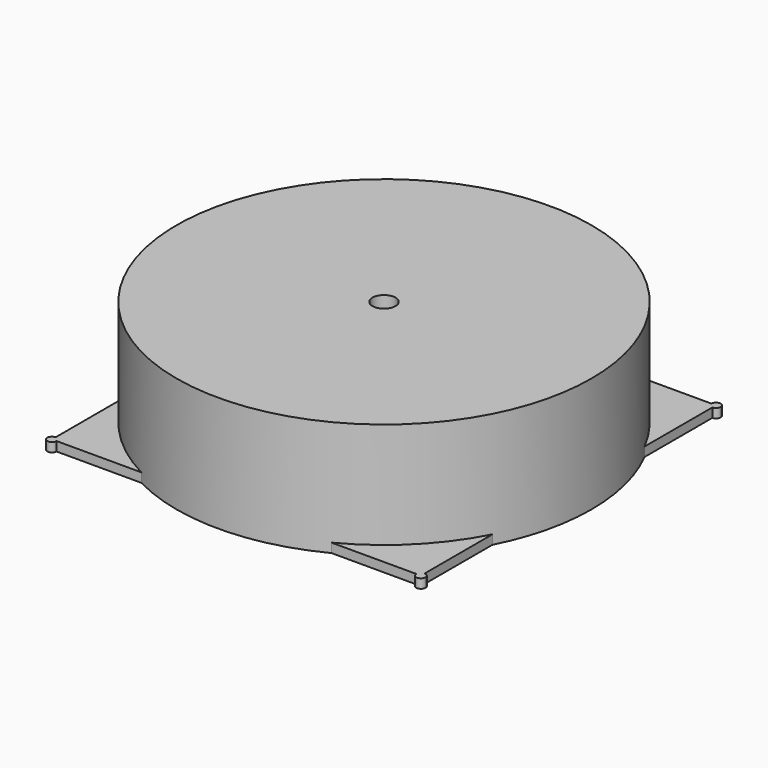
from build123d import *

# Parameters (mm, degrees)
F0_R     = 2.5
F1_DEPTH = 2
F2_DEPTH = 25


# Not quite as in the source:
# - a feature names something its author has since deleted; it is built from what else it names


with BuildPart() as f1:
    # F0 (on Top) → F1 (new body)
    with BuildSketch(Plane.XY):
        with BuildLine():
            ThreePointArc((40, 39), (39.2928932188, 39.2928932188), (39, 40))
            Line((39, 40), (20.6155281281, 40))
            ThreePointArc((20.6155281281, 40), (31.8198051534, 31.8198051534), (40, 20.6155281281))
            Line((40, 20.6155281281), (40, 39))
        make_face()
        with BuildLine():
            ThreePointArc((-40, 20.6155281281), (-31.8198051534, 31.8198051534), (-20.6155281281, 40))
            Line((-20.6155281281, 40), (-39, 40))
            ThreePointArc((-39, 40), (-39.2928932188, 39.2928932188), (-40, 39))
            Line((-40, 39), (-40, 20.6155281281))
        make_face()
        with BuildLine():
            ThreePointArc((-20.6155281281, -40), (-31.8198051534, -31.8198051534), (-40, -20.6155281281))
            Line((-40, -20.6155281281), (-40, -39))
            ThreePointArc((-40, -39), (-39.2928932188, -39.2928932188), (-39, -40))
            Line((-39, -40), (-20.6155281281, -40))
        make_face()
        with BuildLine():
            Line((40, -39), (40, -20.6155281281))
            ThreePointArc((40, -20.6155281281), (31.8198051534, -31.8198051534), (20.6155281281, -40))
            Line((20.6155281281, -40), (39, -40))
            ThreePointArc((39, -40), (39.2928932188, -39.2928932188), (40, -39))
        make_face()
        with BuildLine():
            ThreePointArc((40, 20.6155281281), (31.8198051534, 31.8198051534), (20.6155281281, 40))
            ThreePointArc((20.6155281281, 40), (0, 45), (-20.6155281281, 40))
            ThreePointArc((-20.6155281281, 40), (-31.8198051534, 31.8198051534), (-40, 20.6155281281))
            ThreePointArc((-40, 20.6155281281), (-45, 0), (-40, -20.6155281281))
            ThreePointArc((-40, -20.6155281281), (-31.8198051534, -31.8198051534), (-20.6155281281, -40))
            ThreePointArc((-20.6155281281, -40), (0, -45), (20.6155281281, -40))
            ThreePointArc((20.6155281281, -40), (31.8198051534, -31.8198051534), (40, -20.6155281281))
            ThreePointArc((40, -20.6155281281), (43.7321392113, -10.6066017178), (45, 0))
            ThreePointArc((45, 0), (43.7321392113, 10.6066017178), (40, 20.6155281281))
        make_face()
        Circle(F0_R, mode=Mode.SUBTRACT)
        with BuildLine():
            Line((-40, 40), (-39, 40))
            ThreePointArc((-39, 40), (-40.7071067812, 40.7071067812), (-40, 39))
            Line((-40, 39), (-40, 40))
        make_face()
        with BuildLine():
            ThreePointArc((-40, 39), (-39.2928932188, 39.2928932188), (-39, 40))
            Line((-39, 40), (-40, 40))
            Line((-40, 40), (-40, 39))
        make_face()
        with BuildLine():
            Line((40, 40), (39, 40))
            ThreePointArc((39, 40), (39.2928932188, 39.2928932188), (40, 39))
            Line((40, 39), (40, 40))
        make_face()
        with BuildLine():
            ThreePointArc((40, 39), (40.7071067812, 39.2928932188), (41, 40))
            ThreePointArc((41, 40), (40, 41), (39, 40))
            Line((39, 40), (40, 40))
            Line((40, 40), (40, 39))
        make_face()
        with BuildLine():
            ThreePointArc((41, -40), (40.7071067812, -39.2928932188), (40, -39))
            Line((40, -39), (40, -40))
            Line((40, -40), (39, -40))
            ThreePointArc((39, -40), (40, -41), (41, -40))
        make_face()
        with BuildLine():
            Line((40, -40), (40, -39))
            ThreePointArc((40, -39), (39.2928932188, -39.2928932188), (39, -40))
            Line((39, -40), (40, -40))
        make_face()
        with BuildLine():
            Line((-40, -40), (-40, -39))
            ThreePointArc((-40, -39), (-40.7071067812, -40.7071067812), (-39, -40))
            Line((-39, -40), (-40, -40))
        make_face()
        with BuildLine():
            ThreePointArc((-39, -40), (-39.2928932188, -39.2928932188), (-40, -39))
            Line((-40, -39), (-40, -40))
            Line((-40, -40), (-39, -40))
        make_face()
    extrude(amount=F1_DEPTH)

    # F0 (on Top) → F2 (join)
    with BuildSketch(Plane.XY):
        with BuildLine():
            ThreePointArc((40, 20.6155281281), (31.8198051534, 31.8198051534), (20.6155281281, 40))
            ThreePointArc((20.6155281281, 40), (0, 45), (-20.6155281281, 40))
            ThreePointArc((-20.6155281281, 40), (-31.8198051534, 31.8198051534), (-40, 20.6155281281))
            ThreePointArc((-40, 20.6155281281), (-45, 0), (-40, -20.6155281281))
            ThreePointArc((-40, -20.6155281281), (-31.8198051534, -31.8198051534), (-20.6155281281, -40))
            ThreePointArc((-20.6155281281, -40), (0, -45), (20.6155281281, -40))
            ThreePointArc((20.6155281281, -40), (31.8198051534, -31.8198051534), (40, -20.6155281281))
            ThreePointArc((40, -20.6155281281), (43.7321392113, -10.6066017178), (45, 0))
            ThreePointArc((45, 0), (43.7321392113, 10.6066017178), (40, 20.6155281281))
        make_face()
        Circle(F0_R, mode=Mode.SUBTRACT)
    extrude(amount=F2_DEPTH)


solid = f1.part
